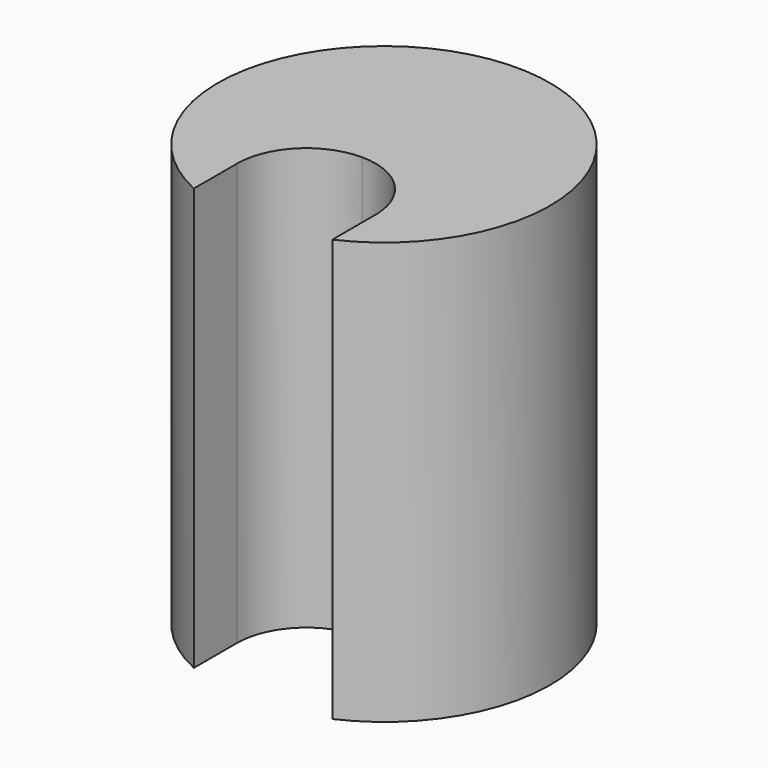
from build123d import *

# Parameters (mm, degrees)
F0_R     = 26.67
F1_DEPTH = 67.7418
F2_W     = 22.225
F2_H     = 22.225
F3_DEPTH = 67.7418
F4_R     = 11.11249
F5_R     = 1.7272
F6_DEPTH = 5.5800505253


# Not quite as in the source:
# - a fillet or chamfer is up to 0.001 mm smaller than in the source, because OpenCascade refuses the exact size


with BuildPart() as f1:
    # F0 (on Top) → F1 (new body)
    with BuildSketch(Plane.XY):
        Circle(F0_R)
    extrude(amount=F1_DEPTH)

    # F2 (on face) → F3 (cut, through all)
    with BuildSketch(Plane.XY.offset(67.7418)):
        with Locations((0, -15.5575)):
            Rectangle(F2_W, F2_H)
    extrude(amount=-F3_DEPTH, mode=Mode.SUBTRACT)

    # F4 (radius 11.1125 in the source; OpenCascade refuses exactly that, so slightly less here)
    f4_edges = [f1.edges().sort_by_distance(p)[0] for p in [
        (11.1125, -4.445, 33.8709),
        (-11.1125, -4.445, 33.8709),
    ]]
    fillet(f4_edges, radius=F4_R)

    # F5 (on Front) → F6 (cut, up to face)
    with BuildSketch(Plane.XZ):
        with Locations((0, 33.8709)):
            Circle(F5_R)
    extrude(amount=F6_DEPTH, mode=Mode.SUBTRACT)


solid = f1.part
